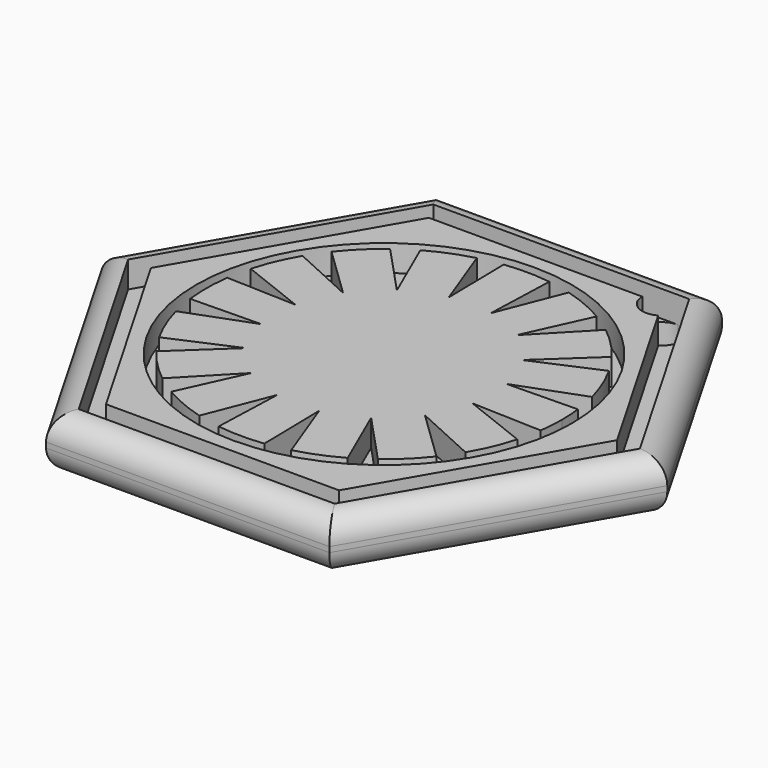
from build123d import *

# Parameters (mm, degrees)
F0_R     = 14.25
F1_DEPTH = 2
F2_DEPTH = 4
F3_R     = 1.79999


# Not quite as in the source:
# - a fillet or chamfer is up to 0.001 mm smaller than in the source, because OpenCascade refuses the exact size


with BuildPart() as f1:
    # F0 (on Top) → F1 (new body)
    with BuildSketch(Plane.XY):
        Polygon((10.75, -18.6195461814), (21.5, 0), (10.75, 18.6195461814), (-10.75, 18.6195461814), (-21.5, 0), (-10.75, -18.6195461814), align=None)
        Polygon((-19.4215390309, 0), (-9.7107695155, 16.8195461814), (8.8447441387, 16.8195461814), (9.7107695155, 16.8195461814), (10.1437822383, 16.069546145), (19.4215390309, 0), (9.7107695155, -16.8195461814), (-9.7107695155, -16.8195461814), align=None, mode=Mode.SUBTRACT)
        with BuildLine():
            ThreePointArc((9.5947441117, 14.0205080757), (8.0947441117, 14.0205080757), (7.3447441117, 15.3195461814))
            Line((7.3447441117, 15.3195461814), (-8.8447441117, 15.3195461814))
            Line((-8.8447441117, 15.3195461814), (-17.6894882233, 0))
            Line((-17.6894882233, 0), (-8.8447441117, -15.3195461814))
            Line((-8.8447441117, -15.3195461814), (8.8447441117, -15.3195461814))
            Line((8.8447441117, -15.3195461814), (17.6894882233, 0))
            Line((17.6894882233, 0), (9.5947441117, 14.0205080757))
        make_face()
        Circle(F0_R, mode=Mode.SUBTRACT)
        Circle(F0_R)
        with BuildLine():
            ThreePointArc((13.3999904986, 1.6401995725), (13.4749744291, 0.8216228664), (13.5, 0))
            ThreePointArc((13.5, 0), (13.4681223582, -0.9271893786), (13.3726399787, -1.85))
            ThreePointArc((13.3726399787, -1.85), (13.2195565752, -2.7373936427), (13.0076541597, -3.6126075434))
            ThreePointArc((13.0076541597, -3.6126075434), (12.4315074952, -5.2638029406), (11.6467440221, -6.826664902))
            ThreePointArc((11.6467440221, -6.826664902), (11.1657225538, -7.5879272435), (10.6350203896, -8.3154279091))
            ThreePointArc((10.6350203896, -8.3154279091), (9.4708451564, -9.6204517577), (8.1477368661, -10.7640319565))
            ThreePointArc((8.1477368661, -10.7640319565), (7.4120084911, -11.2832677061), (6.643301172, -11.7522997553))
            ThreePointArc((6.643301172, -11.7522997553), (5.0683324961, -12.5124740043), (3.4083106317, -13.0626727218))
            ThreePointArc((3.4083106317, -13.0626727218), (2.5298833256, -13.2608329436), (1.6401995725, -13.3999904986))
            ThreePointArc((1.6401995725, -13.3999904986), (-0.1057878423, -13.4995855097), (-1.85, -13.3726399787))
            ThreePointArc((-1.85, -13.3726399787), (-2.7373936427, -13.2195565752), (-3.6126075434, -13.0076541597))
            ThreePointArc((-3.6126075434, -13.0076541597), (-5.2638029406, -12.4315074952), (-6.826664902, -11.6467440221))
            ThreePointArc((-6.826664902, -11.6467440221), (-7.5879272435, -11.1657225538), (-8.3154279091, -10.6350203896))
            ThreePointArc((-8.3154279091, -10.6350203896), (-9.6204517577, -9.4708451564), (-10.7640319565, -8.1477368661))
            ThreePointArc((-10.7640319565, -8.1477368661), (-11.2832677061, -7.4120084911), (-11.7522997553, -6.643301172))
            ThreePointArc((-11.7522997553, -6.643301172), (-12.5124740043, -5.0683324961), (-13.0626727218, -3.4083106317))
            ThreePointArc((-13.0626727218, -3.4083106317), (-13.2608329436, -2.5298833256), (-13.3999904986, -1.6401995725))
            ThreePointArc((-13.3999904986, -1.6401995725), (-13.4995855097, 0.1057878423), (-13.3726399787, 1.85))
            ThreePointArc((-13.3726399787, 1.85), (-13.2195565752, 2.7373936427), (-13.0076541597, 3.6126075434))
            ThreePointArc((-13.0076541597, 3.6126075434), (-12.4315074952, 5.2638029406), (-11.6467440221, 6.826664902))
            ThreePointArc((-11.6467440221, 6.826664902), (-11.1657225538, 7.5879272435), (-10.6350203896, 8.3154279091))
            ThreePointArc((-10.6350203896, 8.3154279091), (-9.4708451564, 9.6204517577), (-8.1477368661, 10.7640319565))
            ThreePointArc((-8.1477368661, 10.7640319565), (-7.4120084911, 11.2832677061), (-6.643301172, 11.7522997553))
            ThreePointArc((-6.643301172, 11.7522997553), (-5.0683324961, 12.5124740043), (-3.4083106317, 13.0626727218))
            ThreePointArc((-3.4083106317, 13.0626727218), (-2.5298833256, 13.2608329436), (-1.6401995725, 13.3999904986))
            ThreePointArc((-1.6401995725, 13.3999904986), (0.1057878423, 13.4995855097), (1.85, 13.3726399787))
            ThreePointArc((1.85, 13.3726399787), (2.7373936427, 13.2195565752), (3.6126075434, 13.0076541597))
            ThreePointArc((3.6126075434, 13.0076541597), (5.2638029406, 12.4315074952), (6.826664902, 11.6467440221))
            ThreePointArc((6.826664902, 11.6467440221), (7.5879272435, 11.1657225538), (8.3154279091, 10.6350203896))
            ThreePointArc((8.3154279091, 10.6350203896), (9.6204517577, 9.4708451564), (10.7640319565, 8.1477368661))
            ThreePointArc((10.7640319565, 8.1477368661), (11.2832677061, 7.4120084911), (11.7522997553, 6.643301172))
            ThreePointArc((11.7522997553, 6.643301172), (12.5124740043, 5.0683324961), (13.0626727218, 3.4083106317))
            ThreePointArc((13.0626727218, 3.4083106317), (13.2608329436, 2.5298833256), (13.3999904986, 1.6401995725))
        make_face(mode=Mode.SUBTRACT)
        with BuildLine():
            ThreePointArc((13.3726399787, -1.85), (13.4681223582, -0.9271893786), (13.5, 0))
            ThreePointArc((13.5, 0), (13.4749744291, 0.8216228664), (13.3999904986, 1.6401995725))
            Line((13.3999904986, 1.6401995725), (8.0735512703, 1.5445602693))
            Line((8.0735512703, 1.5445602693), (13.0626727218, 3.4083106317))
            ThreePointArc((13.0626727218, 3.4083106317), (12.5124740043, 5.0683324961), (11.7522997553, 6.643301172))
            Line((11.7522997553, 6.643301172), (6.867911148, 4.5166019311))
            Line((6.867911148, 4.5166019311), (10.7640319565, 8.1477368661))
            ThreePointArc((10.7640319565, 8.1477368661), (9.6204517577, 9.4708451564), (8.3154279091, 10.6350203896))
            Line((8.3154279091, 10.6350203896), (4.6166938111, 6.8010318919))
            Line((4.6166938111, 6.8010318919), (6.826664902, 11.6467440221))
            ThreePointArc((6.826664902, 11.6467440221), (5.2638029406, 12.4315074952), (3.6126075434, 13.0076541597))
            Line((3.6126075434, 13.0076541597), (1.6626266919, 8.0500663987))
            Line((1.6626266919, 8.0500663987), (1.85, 13.3726399787))
            ThreePointArc((1.85, 13.3726399787), (0.1057878423, 13.4995855097), (-1.6401995725, 13.3999904986))
            Line((-1.6401995725, 13.3999904986), (-1.5445602693, 8.0735512703))
            Line((-1.5445602693, 8.0735512703), (-3.4083106317, 13.0626727218))
            ThreePointArc((-3.4083106317, 13.0626727218), (-5.0683324961, 12.5124740043), (-6.643301172, 11.7522997553))
            Line((-6.643301172, 11.7522997553), (-4.5166019311, 6.867911148))
            Line((-4.5166019311, 6.867911148), (-8.1477368661, 10.7640319565))
            ThreePointArc((-8.1477368661, 10.7640319565), (-9.4708451564, 9.6204517577), (-10.6350203896, 8.3154279091))
            Line((-10.6350203896, 8.3154279091), (-6.8010318919, 4.6166938111))
            Line((-6.8010318919, 4.6166938111), (-11.6467440221, 6.826664902))
            ThreePointArc((-11.6467440221, 6.826664902), (-12.4315074952, 5.2638029406), (-13.0076541597, 3.6126075434))
            Line((-13.0076541597, 3.6126075434), (-8.0500663987, 1.6626266919))
            Line((-8.0500663987, 1.6626266919), (-13.3726399787, 1.85))
            ThreePointArc((-13.3726399787, 1.85), (-13.4995855097, 0.1057878423), (-13.3999904986, -1.6401995725))
            Line((-13.3999904986, -1.6401995725), (-8.0735512703, -1.5445602693))
            Line((-8.0735512703, -1.5445602693), (-13.0626727218, -3.4083106317))
            ThreePointArc((-13.0626727218, -3.4083106317), (-12.5124740043, -5.0683324961), (-11.7522997553, -6.643301172))
            Line((-11.7522997553, -6.643301172), (-6.867911148, -4.5166019311))
            Line((-6.867911148, -4.5166019311), (-10.7640319565, -8.1477368661))
            ThreePointArc((-10.7640319565, -8.1477368661), (-9.6204517577, -9.4708451564), (-8.3154279091, -10.6350203896))
            Line((-8.3154279091, -10.6350203896), (-4.6166938111, -6.8010318919))
            Line((-4.6166938111, -6.8010318919), (-6.826664902, -11.6467440221))
            ThreePointArc((-6.826664902, -11.6467440221), (-5.2638029406, -12.4315074952), (-3.6126075434, -13.0076541597))
            Line((-3.6126075434, -13.0076541597), (-1.6626266919, -8.0500663987))
            Line((-1.6626266919, -8.0500663987), (-1.85, -13.3726399787))
            ThreePointArc((-1.85, -13.3726399787), (-0.1057878423, -13.4995855097), (1.6401995725, -13.3999904986))
            Line((1.6401995725, -13.3999904986), (1.5445602693, -8.0735512703))
            Line((1.5445602693, -8.0735512703), (3.4083106317, -13.0626727218))
            ThreePointArc((3.4083106317, -13.0626727218), (5.0683324961, -12.5124740043), (6.643301172, -11.7522997553))
            Line((6.643301172, -11.7522997553), (4.5166019311, -6.867911148))
            Line((4.5166019311, -6.867911148), (8.1477368661, -10.7640319565))
            ThreePointArc((8.1477368661, -10.7640319565), (9.4708451564, -9.6204517577), (10.6350203896, -8.3154279091))
            Line((10.6350203896, -8.3154279091), (6.8010318919, -4.6166938111))
            Line((6.8010318919, -4.6166938111), (11.6467440221, -6.826664902))
            ThreePointArc((11.6467440221, -6.826664902), (12.4315074952, -5.2638029406), (13.0076541597, -3.6126075434))
            Line((13.0076541597, -3.6126075434), (8.0500663987, -1.6626266919))
            Line((8.0500663987, -1.6626266919), (13.3726399787, -1.85))
        make_face()
        with BuildLine():
            Line((8.8447441387, 16.8195461814), (-9.7107695155, 16.8195461814))
            Line((-9.7107695155, 16.8195461814), (-19.4215390309, 0))
            Line((-19.4215390309, 0), (-9.7107695155, -16.8195461814))
            Line((-9.7107695155, -16.8195461814), (9.7107695155, -16.8195461814))
            Line((9.7107695155, -16.8195461814), (19.4215390309, 0))
            Line((19.4215390309, 0), (10.1437822383, 16.069546145))
            ThreePointArc((10.1437822383, 16.069546145), (10.2936328565, 15.7077747288), (10.3447441117, 15.3195461814))
            ThreePointArc((10.3447441117, 15.3195461814), (10.1437822174, 14.5695461814), (9.5947441117, 14.0205080757))
            Line((9.5947441117, 14.0205080757), (17.6894882233, 0))
            Line((17.6894882233, 0), (8.8447441117, -15.3195461814))
            Line((8.8447441117, -15.3195461814), (-8.8447441117, -15.3195461814))
            Line((-8.8447441117, -15.3195461814), (-17.6894882233, 0))
            Line((-17.6894882233, 0), (-8.8447441117, 15.3195461814))
            Line((-8.8447441117, 15.3195461814), (7.3447441117, 15.3195461814))
            ThreePointArc((7.3447441117, 15.3195461814), (7.7840839495, 16.3802063627), (8.8447441387, 16.8195461814))
        make_face()
        with BuildLine():
            ThreePointArc((-11.7522997553, -6.643301172), (-11.2832677061, -7.4120084911), (-10.7640319565, -8.1477368661))
            Line((-10.7640319565, -8.1477368661), (-6.867911148, -4.5166019311))
            Line((-6.867911148, -4.5166019311), (-11.7522997553, -6.643301172))
        make_face()
        with BuildLine():
            ThreePointArc((-8.3154279091, -10.6350203896), (-7.5879272435, -11.1657225538), (-6.826664902, -11.6467440221))
            Line((-6.826664902, -11.6467440221), (-4.6166938111, -6.8010318919))
            Line((-4.6166938111, -6.8010318919), (-8.3154279091, -10.6350203896))
        make_face()
        with BuildLine():
            ThreePointArc((-3.6126075434, -13.0076541597), (-2.7373936427, -13.2195565752), (-1.85, -13.3726399787))
            Line((-1.85, -13.3726399787), (-1.6626266919, -8.0500663987))
            Line((-1.6626266919, -8.0500663987), (-3.6126075434, -13.0076541597))
        make_face()
        with BuildLine():
            ThreePointArc((1.6401995725, -13.3999904986), (2.5298833256, -13.2608329436), (3.4083106317, -13.0626727218))
            Line((3.4083106317, -13.0626727218), (1.5445602693, -8.0735512703))
            Line((1.5445602693, -8.0735512703), (1.6401995725, -13.3999904986))
        make_face()
        with BuildLine():
            ThreePointArc((6.643301172, -11.7522997553), (7.4120084911, -11.2832677061), (8.1477368661, -10.7640319565))
            Line((8.1477368661, -10.7640319565), (4.5166019311, -6.867911148))
            Line((4.5166019311, -6.867911148), (6.643301172, -11.7522997553))
        make_face()
        with BuildLine():
            ThreePointArc((10.6350203896, -8.3154279091), (11.1657225538, -7.5879272435), (11.6467440221, -6.826664902))
            Line((11.6467440221, -6.826664902), (6.8010318919, -4.6166938111))
            Line((6.8010318919, -4.6166938111), (10.6350203896, -8.3154279091))
        make_face()
        with BuildLine():
            ThreePointArc((13.0076541597, -3.6126075434), (13.2195565752, -2.7373936427), (13.3726399787, -1.85))
            Line((13.3726399787, -1.85), (8.0500663987, -1.6626266919))
            Line((8.0500663987, -1.6626266919), (13.0076541597, -3.6126075434))
        make_face()
        with BuildLine():
            Line((8.0735512703, 1.5445602693), (13.3999904986, 1.6401995725))
            ThreePointArc((13.3999904986, 1.6401995725), (13.2608329436, 2.5298833256), (13.0626727218, 3.4083106317))
            Line((13.0626727218, 3.4083106317), (8.0735512703, 1.5445602693))
        make_face()
        with BuildLine():
            Line((6.867911148, 4.5166019311), (11.7522997553, 6.643301172))
            ThreePointArc((11.7522997553, 6.643301172), (11.2832677061, 7.4120084911), (10.7640319565, 8.1477368661))
            Line((10.7640319565, 8.1477368661), (6.867911148, 4.5166019311))
        make_face()
        with BuildLine():
            Line((4.6166938111, 6.8010318919), (8.3154279091, 10.6350203896))
            ThreePointArc((8.3154279091, 10.6350203896), (7.5879272435, 11.1657225538), (6.826664902, 11.6467440221))
            Line((6.826664902, 11.6467440221), (4.6166938111, 6.8010318919))
        make_face()
        with BuildLine():
            Line((1.6626266919, 8.0500663987), (3.6126075434, 13.0076541597))
            ThreePointArc((3.6126075434, 13.0076541597), (2.7373936427, 13.2195565752), (1.85, 13.3726399787))
            Line((1.85, 13.3726399787), (1.6626266919, 8.0500663987))
        make_face()
        with BuildLine():
            Line((-1.5445602693, 8.0735512703), (-1.6401995725, 13.3999904986))
            ThreePointArc((-1.6401995725, 13.3999904986), (-2.5298833256, 13.2608329436), (-3.4083106317, 13.0626727218))
            Line((-3.4083106317, 13.0626727218), (-1.5445602693, 8.0735512703))
        make_face()
        with BuildLine():
            Line((-4.5166019311, 6.867911148), (-6.643301172, 11.7522997553))
            ThreePointArc((-6.643301172, 11.7522997553), (-7.4120084911, 11.2832677061), (-8.1477368661, 10.7640319565))
            Line((-8.1477368661, 10.7640319565), (-4.5166019311, 6.867911148))
        make_face()
        with BuildLine():
            Line((-6.8010318919, 4.6166938111), (-10.6350203896, 8.3154279091))
            ThreePointArc((-10.6350203896, 8.3154279091), (-11.1657225538, 7.5879272435), (-11.6467440221, 6.826664902))
            Line((-11.6467440221, 6.826664902), (-6.8010318919, 4.6166938111))
        make_face()
        with BuildLine():
            Line((-8.0500663987, 1.6626266919), (-13.0076541597, 3.6126075434))
            ThreePointArc((-13.0076541597, 3.6126075434), (-13.2195565752, 2.7373936427), (-13.3726399787, 1.85))
            Line((-13.3726399787, 1.85), (-8.0500663987, 1.6626266919))
        make_face()
        with BuildLine():
            ThreePointArc((-13.3999904986, -1.6401995725), (-13.2608329436, -2.5298833256), (-13.0626727218, -3.4083106317))
            Line((-13.0626727218, -3.4083106317), (-8.0735512703, -1.5445602693))
            Line((-8.0735512703, -1.5445602693), (-13.3999904986, -1.6401995725))
        make_face()
    extrude(amount=F1_DEPTH)

    # F0 (on Top) → F2 (join)
    with BuildSketch(Plane.XY):
        Polygon((10.75, -18.6195461814), (21.5, 0), (10.75, 18.6195461814), (-10.75, 18.6195461814), (-21.5, 0), (-10.75, -18.6195461814), align=None)
        Polygon((-19.4215390309, 0), (-9.7107695155, 16.8195461814), (8.8447441387, 16.8195461814), (9.7107695155, 16.8195461814), (10.1437822383, 16.069546145), (19.4215390309, 0), (9.7107695155, -16.8195461814), (-9.7107695155, -16.8195461814), align=None, mode=Mode.SUBTRACT)
        with BuildLine():
            ThreePointArc((9.5947441117, 14.0205080757), (8.0947441117, 14.0205080757), (7.3447441117, 15.3195461814))
            Line((7.3447441117, 15.3195461814), (-8.8447441117, 15.3195461814))
            Line((-8.8447441117, 15.3195461814), (-17.6894882233, 0))
            Line((-17.6894882233, 0), (-8.8447441117, -15.3195461814))
            Line((-8.8447441117, -15.3195461814), (8.8447441117, -15.3195461814))
            Line((8.8447441117, -15.3195461814), (17.6894882233, 0))
            Line((17.6894882233, 0), (9.5947441117, 14.0205080757))
        make_face()
        Circle(F0_R, mode=Mode.SUBTRACT)
        with BuildLine():
            ThreePointArc((13.3726399787, -1.85), (13.4681223582, -0.9271893786), (13.5, 0))
            ThreePointArc((13.5, 0), (13.4749744291, 0.8216228664), (13.3999904986, 1.6401995725))
            Line((13.3999904986, 1.6401995725), (8.0735512703, 1.5445602693))
            Line((8.0735512703, 1.5445602693), (13.0626727218, 3.4083106317))
            ThreePointArc((13.0626727218, 3.4083106317), (12.5124740043, 5.0683324961), (11.7522997553, 6.643301172))
            Line((11.7522997553, 6.643301172), (6.867911148, 4.5166019311))
            Line((6.867911148, 4.5166019311), (10.7640319565, 8.1477368661))
            ThreePointArc((10.7640319565, 8.1477368661), (9.6204517577, 9.4708451564), (8.3154279091, 10.6350203896))
            Line((8.3154279091, 10.6350203896), (4.6166938111, 6.8010318919))
            Line((4.6166938111, 6.8010318919), (6.826664902, 11.6467440221))
            ThreePointArc((6.826664902, 11.6467440221), (5.2638029406, 12.4315074952), (3.6126075434, 13.0076541597))
            Line((3.6126075434, 13.0076541597), (1.6626266919, 8.0500663987))
            Line((1.6626266919, 8.0500663987), (1.85, 13.3726399787))
            ThreePointArc((1.85, 13.3726399787), (0.1057878423, 13.4995855097), (-1.6401995725, 13.3999904986))
            Line((-1.6401995725, 13.3999904986), (-1.5445602693, 8.0735512703))
            Line((-1.5445602693, 8.0735512703), (-3.4083106317, 13.0626727218))
            ThreePointArc((-3.4083106317, 13.0626727218), (-5.0683324961, 12.5124740043), (-6.643301172, 11.7522997553))
            Line((-6.643301172, 11.7522997553), (-4.5166019311, 6.867911148))
            Line((-4.5166019311, 6.867911148), (-8.1477368661, 10.7640319565))
            ThreePointArc((-8.1477368661, 10.7640319565), (-9.4708451564, 9.6204517577), (-10.6350203896, 8.3154279091))
            Line((-10.6350203896, 8.3154279091), (-6.8010318919, 4.6166938111))
            Line((-6.8010318919, 4.6166938111), (-11.6467440221, 6.826664902))
            ThreePointArc((-11.6467440221, 6.826664902), (-12.4315074952, 5.2638029406), (-13.0076541597, 3.6126075434))
            Line((-13.0076541597, 3.6126075434), (-8.0500663987, 1.6626266919))
            Line((-8.0500663987, 1.6626266919), (-13.3726399787, 1.85))
            ThreePointArc((-13.3726399787, 1.85), (-13.4995855097, 0.1057878423), (-13.3999904986, -1.6401995725))
            Line((-13.3999904986, -1.6401995725), (-8.0735512703, -1.5445602693))
            Line((-8.0735512703, -1.5445602693), (-13.0626727218, -3.4083106317))
            ThreePointArc((-13.0626727218, -3.4083106317), (-12.5124740043, -5.0683324961), (-11.7522997553, -6.643301172))
            Line((-11.7522997553, -6.643301172), (-6.867911148, -4.5166019311))
            Line((-6.867911148, -4.5166019311), (-10.7640319565, -8.1477368661))
            ThreePointArc((-10.7640319565, -8.1477368661), (-9.6204517577, -9.4708451564), (-8.3154279091, -10.6350203896))
            Line((-8.3154279091, -10.6350203896), (-4.6166938111, -6.8010318919))
            Line((-4.6166938111, -6.8010318919), (-6.826664902, -11.6467440221))
            ThreePointArc((-6.826664902, -11.6467440221), (-5.2638029406, -12.4315074952), (-3.6126075434, -13.0076541597))
            Line((-3.6126075434, -13.0076541597), (-1.6626266919, -8.0500663987))
            Line((-1.6626266919, -8.0500663987), (-1.85, -13.3726399787))
            ThreePointArc((-1.85, -13.3726399787), (-0.1057878423, -13.4995855097), (1.6401995725, -13.3999904986))
            Line((1.6401995725, -13.3999904986), (1.5445602693, -8.0735512703))
            Line((1.5445602693, -8.0735512703), (3.4083106317, -13.0626727218))
            ThreePointArc((3.4083106317, -13.0626727218), (5.0683324961, -12.5124740043), (6.643301172, -11.7522997553))
            Line((6.643301172, -11.7522997553), (4.5166019311, -6.867911148))
            Line((4.5166019311, -6.867911148), (8.1477368661, -10.7640319565))
            ThreePointArc((8.1477368661, -10.7640319565), (9.4708451564, -9.6204517577), (10.6350203896, -8.3154279091))
            Line((10.6350203896, -8.3154279091), (6.8010318919, -4.6166938111))
            Line((6.8010318919, -4.6166938111), (11.6467440221, -6.826664902))
            ThreePointArc((11.6467440221, -6.826664902), (12.4315074952, -5.2638029406), (13.0076541597, -3.6126075434))
            Line((13.0076541597, -3.6126075434), (8.0500663987, -1.6626266919))
            Line((8.0500663987, -1.6626266919), (13.3726399787, -1.85))
        make_face()
    extrude(amount=F2_DEPTH)

    # F3 (radius 1.8 in the source; OpenCascade refuses exactly that, so slightly less here)
    f3_edges = [f1.edges().sort_by_distance(p)[0] for p in [
        (-16.125, -9.309773, 4),
        (-16.125, 9.309773, 4),
        (0, 18.619546, 4),
        (16.125, 9.309773, 4),
        (16.125, -9.309773, 4),
        (0, -18.619546, 4),
        (16.125, -9.309773, 0),
        (0, -18.619546, 0),
        (16.125, 9.309773, 0),
        (0, 18.619546, 0),
        (-16.125, 9.309773, 0),
        (-16.125, -9.309773, 0),
    ]]
    fillet(f3_edges, radius=F3_R)


solid = f1.part
